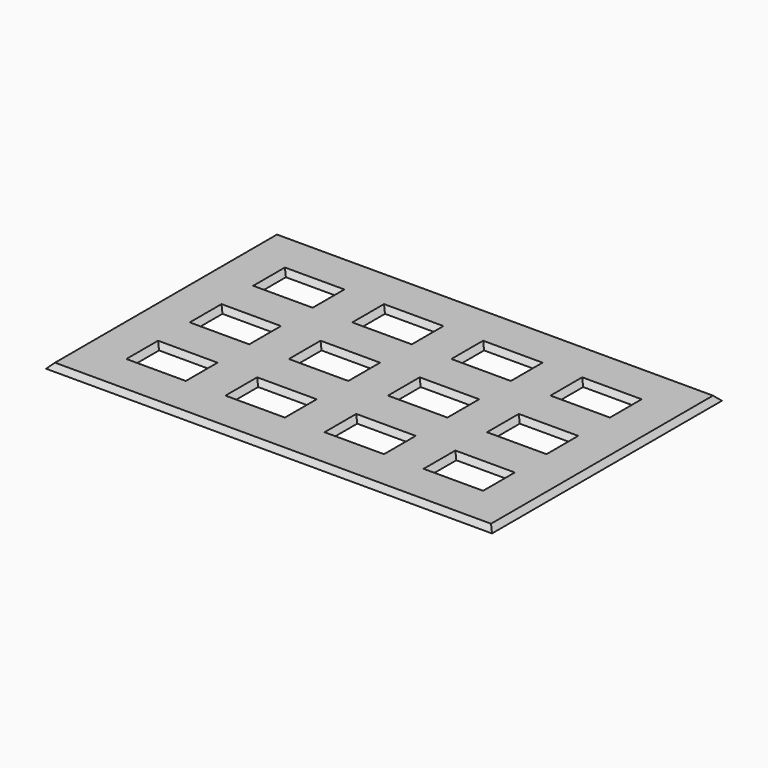
from build123d import *

# Parameters (mm, degrees)
F0_W     = 90
F0_H     = 58
F0_W_2   = 10
F0_H_2   = 6
F1_DEPTH = 1
F2_SIZE  = 0.99999


# Not quite as in the source:
# - a fillet or chamfer is up to 0.001 mm smaller than in the source, because OpenCascade refuses the exact size


with BuildPart() as f1:
    # F0 (on Top) → F1 (new body)
    with BuildSketch(Plane.XY):
        with Locations((-5, -4)):
            Rectangle(F0_W, F0_H)
        with Locations((-35, -20)):
            Rectangle(F0_W_2, F0_H_2, mode=Mode.SUBTRACT)
        with Locations((-15, -20)):
            Rectangle(F0_W_2, F0_H_2, mode=Mode.SUBTRACT)
        with Locations((5, -20)):
            Rectangle(F0_W_2, F0_H_2, mode=Mode.SUBTRACT)
        with Locations((25, -20)):
            Rectangle(F0_W_2, F0_H_2, mode=Mode.SUBTRACT)
        with Locations((-35, -4)):
            Rectangle(F0_W_2, F0_H_2, mode=Mode.SUBTRACT)
        with Locations((-15, -4)):
            Rectangle(F0_W_2, F0_H_2, mode=Mode.SUBTRACT)
        with Locations((-35, 12)):
            Rectangle(F0_W_2, F0_H_2, mode=Mode.SUBTRACT)
        with Locations((-15, 12)):
            Rectangle(F0_W_2, F0_H_2, mode=Mode.SUBTRACT)
        with Locations((5, -4)):
            Rectangle(F0_W_2, F0_H_2, mode=Mode.SUBTRACT)
        with Locations((25, -4)):
            Rectangle(F0_W_2, F0_H_2, mode=Mode.SUBTRACT)
        with Locations((5, 12)):
            Rectangle(F0_W_2, F0_H_2, mode=Mode.SUBTRACT)
        with Locations((25, 12)):
            Rectangle(F0_W_2, F0_H_2, mode=Mode.SUBTRACT)
    extrude(amount=F1_DEPTH)

    # F2 (size 1 in the source; OpenCascade refuses exactly that, so slightly less here)
    f2_edges = [f1.edges().sort_by_distance(p)[0] for p in [
        (-35, 15, 1),
        (-40, 12, 1),
        (-35, 9, 1),
        (-30, 12, 1),
        (-30, -4, 1),
        (-35, -7, 1),
        (-35, -1, 1),
        (-40, -4, 1),
        (-35, -17, 1),
        (-40, -20, 1),
        (-35, -23, 1),
        (-30, -20, 1),
        (-5, 25, 1),
        (-50, -4, 1),
        (-5, -33, 1),
        (40, -4, 1),
        (-20, -20, 1),
        (-15, -17, 1),
        (-10, -20, 1),
        (-15, -23, 1),
        (5, -23, 1),
        (0, -20, 1),
        (5, -17, 1),
        (10, -20, 1),
        (25, -23, 1),
        (20, -20, 1),
        (25, -17, 1),
        (30, -20, 1),
        (-20, -4, 1),
        (-15, -1, 1),
        (-10, -4, 1),
        (-15, -7, 1),
        (-20, 12, 1),
        (-15, 15, 1),
        (-10, 12, 1),
        (-15, 9, 1),
        (5, -7, 1),
        (0, -4, 1),
        (5, -1, 1),
        (10, -4, 1),
        (25, -7, 1),
        (20, -4, 1),
        (25, -1, 1),
        (30, -4, 1),
        (0, 12, 1),
        (5, 15, 1),
        (10, 12, 1),
        (5, 9, 1),
        (25, 9, 1),
        (20, 12, 1),
        (25, 15, 1),
        (30, 12, 1),
    ]]
    chamfer(f2_edges, length=F2_SIZE)


solid = f1.part
